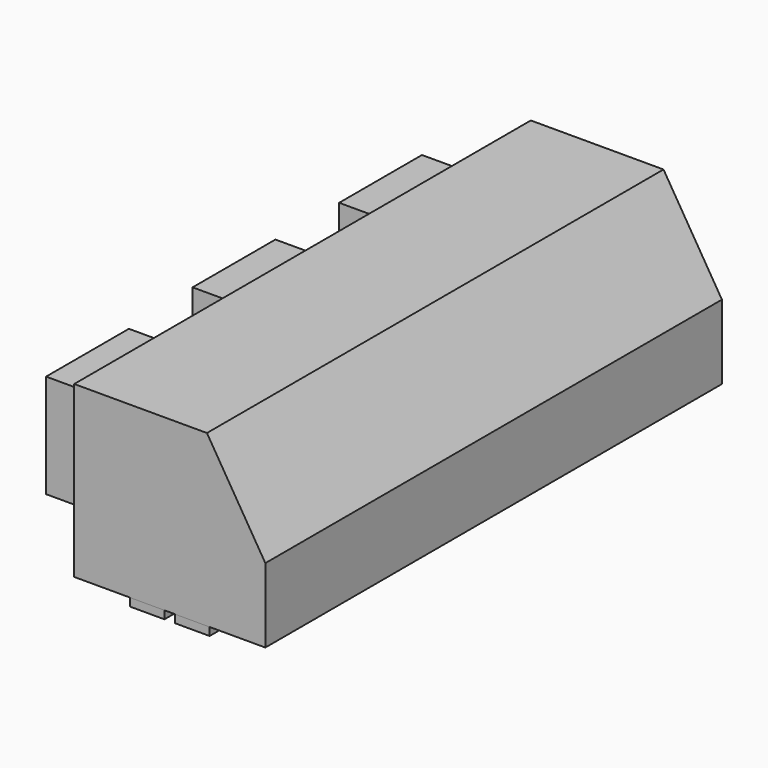
from build123d import *

# Parameters (mm, degrees)
F1_DEPTH = 215
F2_W     = 39
F2_H     = 39
F3_DEPTH = 13
F4_W     = 39
F4_H     = 39
F5_DEPTH = 13
F6_W     = 13
F6_H     = 215
F7_DEPTH = 3
F6_H_2   = 165


with BuildPart() as f1:
    # F0 (on Front) → F1 (new body)
    with BuildSketch(Plane.XZ):
        Polygon((0, 64), (0, 0), (72, 0), (72, 28), (50, 64), align=None)
    extrude(amount=-F1_DEPTH)

    # F2 (on face) → F3 (join)
    with BuildSketch(Plane(origin=(0, 0, 0), x_dir=(0, -1, 0), z_dir=(-1, 0, 0))):
        with Locations((-22.5, 41.5)):
            Rectangle(F2_W, F2_H)
        Polygon((-26.9211616751, 58), (-18.0788383249, 58), (-10.4211616751, 53.5788383249), (-6, 45.9211616751), (-6, 37.0788383249), (-10.4211616751, 29.4211616751), (-18.0788383249, 25), (-26.9211616751, 25), (-34.5788383249, 29.4211616751), (-39, 37.0788383249), (-39, 45.9211616751), (-34.5788383249, 53.5788383249), align=None, mode=Mode.SUBTRACT)
    extrude(amount=F3_DEPTH)

    # F4 (on face) → F5 (join, through all)
    with BuildSketch(Plane(origin=(0, 0, 0), x_dir=(0, -1, 0), z_dir=(-1, 0, 0))):
        with Locations((-91.5, 43.0553856975)):
            Rectangle(F4_W, F4_H)
        Polygon((-95.9211616751, 59.5553856975), (-87.0788383249, 59.5553856975), (-79.4211616751, 55.1342240224), (-75, 47.4765473726), (-75, 38.6342240224), (-79.4211616751, 30.9765473726), (-87.0788383249, 26.5553856975), (-95.9211616751, 26.5553856975), (-103.5788383249, 30.9765473726), (-108, 38.6342240224), (-108, 47.4765473726), (-103.5788383249, 55.1342240224), align=None, mode=Mode.SUBTRACT)
        with Locations((-160.5, 43.0450536048)):
            Rectangle(F4_W, F4_H)
        Polygon((-164.9211616751, 59.5450536048), (-156.0788383249, 59.5450536048), (-148.4211616751, 55.1238919297), (-144, 47.4662152799), (-144, 38.6238919297), (-148.4211616751, 30.9662152799), (-156.0788383249, 26.5450536048), (-164.9211616751, 26.5450536048), (-172.5788383249, 30.9662152799), (-177, 38.6238919297), (-177, 47.4662152799), (-172.5788383249, 55.1238919297), align=None, mode=Mode.SUBTRACT)
    extrude(amount=F5_DEPTH)


with BuildPart() as f7:
    # F6 (on face) → F7 (new body)
    with BuildSketch(Plane(origin=(0, 0, 0), x_dir=(1, 0, 0), z_dir=(0, 0, -1))):
        with Locations((27.5, -107.5)):
            Rectangle(F6_W, F6_H)
    extrude(amount=F7_DEPTH)


with BuildPart() as f7b:
    # F6 (on face) → F7, piece 2 (new body)
    with BuildSketch(Plane(origin=(0, 0, 0), x_dir=(1, 0, 0), z_dir=(0, 0, -1))):
        with Locations((44.5, -107.5)):
            Rectangle(F6_W, F6_H)
    extrude(amount=F7_DEPTH)


with BuildPart() as f7c:
    # F6 (on face) → F7, piece 3 (new body)
    with BuildSketch(Plane(origin=(0, 0, 0), x_dir=(1, 0, 0), z_dir=(0, 0, -1))):
        with Locations((10.5, -107.5)):
            Rectangle(F6_W, F6_H_2)
    extrude(amount=F7_DEPTH)


with BuildPart() as f7d:
    # F6 (on face) → F7, piece 4 (new body)
    with BuildSketch(Plane(origin=(0, 0, 0), x_dir=(1, 0, 0), z_dir=(0, 0, -1))):
        with Locations((61.5, -107.5)):
            Rectangle(F6_W, F6_H_2)
    extrude(amount=F7_DEPTH)


solid = Compound([f1.part, f7.part, f7b.part, f7c.part, f7d.part])
